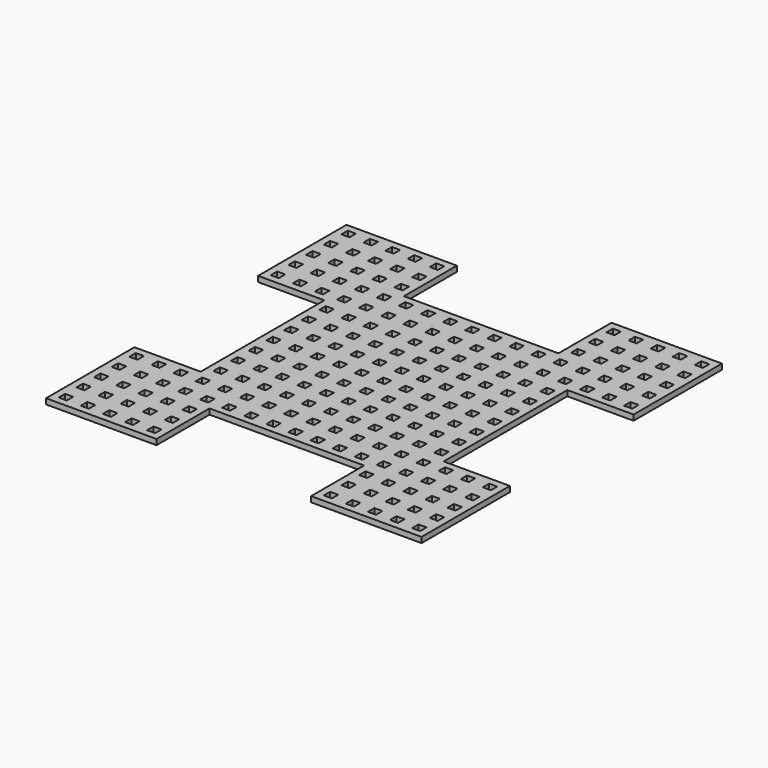
from build123d import *

# Parameters (mm, degrees)
F0_W     = 4.6228
F0_H     = 4.6228
F1_DEPTH = 3.175


# Not quite as in the source:
# - a length typed as a fraction of an inch, garbled in the dataset ("3 / 203.2 mm" for 3/8 in), is restored


with BuildPart() as f1:
    # F0 (on Top) → F1 (new body)
    with BuildSketch(Plane.XY):
        Polygon((114.3, 101.6), (101.6, 101.6), (50.8, 101.6), (50.8, 63.5), (-38.1, 63.5), (-38.1, 101.6), (-95.25, 101.6), (-101.6, 101.6), (-101.6, 95.25), (-101.6, 38.1), (-63.5, 38.1), (-63.5, -50.8), (-101.6, -50.8), (-101.6, -114.3), (-38.1, -114.3), (-38.1, -76.2), (50.8, -76.2), (50.8, -114.3), (114.3, -114.3), (114.3, -50.8), (76.2, -50.8), (76.2, 38.1), (114.3, 38.1), align=None)
        with Locations((-95.25, -107.95)):
            Rectangle(F0_W, F0_H, mode=Mode.SUBTRACT)
        with Locations((-82.55, -107.95)):
            Rectangle(F0_W, F0_H, mode=Mode.SUBTRACT)
        with Locations((-95.25, -95.25)):
            Rectangle(F0_W, F0_H, mode=Mode.SUBTRACT)
        with Locations((-82.55, -95.25)):
            Rectangle(F0_W, F0_H, mode=Mode.SUBTRACT)
        with Locations((-69.85, -107.95)):
            Rectangle(F0_W, F0_H, mode=Mode.SUBTRACT)
        with Locations((-57.15, -107.95)):
            Rectangle(F0_W, F0_H, mode=Mode.SUBTRACT)
        with Locations((-69.85, -95.25)):
            Rectangle(F0_W, F0_H, mode=Mode.SUBTRACT)
        with Locations((-57.15, -95.25)):
            Rectangle(F0_W, F0_H, mode=Mode.SUBTRACT)
        with Locations((-95.25, -82.55)):
            Rectangle(F0_W, F0_H, mode=Mode.SUBTRACT)
        with Locations((-82.55, -82.55)):
            Rectangle(F0_W, F0_H, mode=Mode.SUBTRACT)
        with Locations((-95.25, -69.85)):
            Rectangle(F0_W, F0_H, mode=Mode.SUBTRACT)
        with Locations((-82.55, -69.85)):
            Rectangle(F0_W, F0_H, mode=Mode.SUBTRACT)
        with Locations((-69.85, -82.55)):
            Rectangle(F0_W, F0_H, mode=Mode.SUBTRACT)
        with Locations((-57.15, -82.55)):
            Rectangle(F0_W, F0_H, mode=Mode.SUBTRACT)
        with Locations((-69.85, -69.85)):
            Rectangle(F0_W, F0_H, mode=Mode.SUBTRACT)
        with Locations((-57.15, -69.85)):
            Rectangle(F0_W, F0_H, mode=Mode.SUBTRACT)
        with Locations((-44.45, -107.95)):
            Rectangle(F0_W, F0_H, mode=Mode.SUBTRACT)
        with Locations((-44.45, -95.25)):
            Rectangle(F0_W, F0_H, mode=Mode.SUBTRACT)
        with Locations((-44.45, -82.55)):
            Rectangle(F0_W, F0_H, mode=Mode.SUBTRACT)
        with Locations((-44.45, -69.85)):
            Rectangle(F0_W, F0_H, mode=Mode.SUBTRACT)
        with Locations((-31.75, -69.85)):
            Rectangle(F0_W, F0_H, mode=Mode.SUBTRACT)
        with Locations((-19.05, -69.85)):
            Rectangle(F0_W, F0_H, mode=Mode.SUBTRACT)
        with Locations((-6.35, -69.85)):
            Rectangle(F0_W, F0_H, mode=Mode.SUBTRACT)
        with Locations((-95.25, -57.15)):
            Rectangle(F0_W, F0_H, mode=Mode.SUBTRACT)
        with Locations((-82.55, -57.15)):
            Rectangle(F0_W, F0_H, mode=Mode.SUBTRACT)
        with Locations((-69.85, -57.15)):
            Rectangle(F0_W, F0_H, mode=Mode.SUBTRACT)
        with Locations((-57.15, -57.15)):
            Rectangle(F0_W, F0_H, mode=Mode.SUBTRACT)
        with Locations((-57.15, -44.45)):
            Rectangle(F0_W, F0_H, mode=Mode.SUBTRACT)
        with Locations((-57.15, -31.75)):
            Rectangle(F0_W, F0_H, mode=Mode.SUBTRACT)
        with Locations((-57.15, -19.05)):
            Rectangle(F0_W, F0_H, mode=Mode.SUBTRACT)
        with Locations((-44.45, -57.15)):
            Rectangle(F0_W, F0_H, mode=Mode.SUBTRACT)
        with Locations((-31.75, -57.15)):
            Rectangle(F0_W, F0_H, mode=Mode.SUBTRACT)
        with Locations((-44.45, -44.45)):
            Rectangle(F0_W, F0_H, mode=Mode.SUBTRACT)
        with Locations((-31.75, -44.45)):
            Rectangle(F0_W, F0_H, mode=Mode.SUBTRACT)
        with Locations((-19.05, -57.15)):
            Rectangle(F0_W, F0_H, mode=Mode.SUBTRACT)
        with Locations((-6.35, -57.15)):
            Rectangle(F0_W, F0_H, mode=Mode.SUBTRACT)
        with Locations((-19.05, -44.45)):
            Rectangle(F0_W, F0_H, mode=Mode.SUBTRACT)
        with Locations((-6.35, -44.45)):
            Rectangle(F0_W, F0_H, mode=Mode.SUBTRACT)
        with Locations((-44.45, -31.75)):
            Rectangle(F0_W, F0_H, mode=Mode.SUBTRACT)
        with Locations((-31.75, -31.75)):
            Rectangle(F0_W, F0_H, mode=Mode.SUBTRACT)
        with Locations((-44.45, -19.05)):
            Rectangle(F0_W, F0_H, mode=Mode.SUBTRACT)
        with Locations((-31.75, -19.05)):
            Rectangle(F0_W, F0_H, mode=Mode.SUBTRACT)
        with Locations((-19.05, -31.75)):
            Rectangle(F0_W, F0_H, mode=Mode.SUBTRACT)
        with Locations((-6.35, -31.75)):
            Rectangle(F0_W, F0_H, mode=Mode.SUBTRACT)
        with Locations((-19.05, -19.05)):
            Rectangle(F0_W, F0_H, mode=Mode.SUBTRACT)
        with Locations((-6.35, -19.05)):
            Rectangle(F0_W, F0_H, mode=Mode.SUBTRACT)
        with Locations((57.15, -107.95)):
            Rectangle(F0_W, F0_H, mode=Mode.SUBTRACT)
        with Locations((57.15, -95.25)):
            Rectangle(F0_W, F0_H, mode=Mode.SUBTRACT)
        with Locations((6.35, -69.85)):
            Rectangle(F0_W, F0_H, mode=Mode.SUBTRACT)
        with Locations((19.05, -69.85)):
            Rectangle(F0_W, F0_H, mode=Mode.SUBTRACT)
        with Locations((31.75, -69.85)):
            Rectangle(F0_W, F0_H, mode=Mode.SUBTRACT)
        with Locations((57.15, -82.55)):
            Rectangle(F0_W, F0_H, mode=Mode.SUBTRACT)
        with Locations((44.45, -69.85)):
            Rectangle(F0_W, F0_H, mode=Mode.SUBTRACT)
        with Locations((57.15, -69.85)):
            Rectangle(F0_W, F0_H, mode=Mode.SUBTRACT)
        with Locations((69.85, -107.95)):
            Rectangle(F0_W, F0_H, mode=Mode.SUBTRACT)
        with Locations((82.55, -107.95)):
            Rectangle(F0_W, F0_H, mode=Mode.SUBTRACT)
        with Locations((69.85, -95.25)):
            Rectangle(F0_W, F0_H, mode=Mode.SUBTRACT)
        with Locations((82.55, -95.25)):
            Rectangle(F0_W, F0_H, mode=Mode.SUBTRACT)
        with Locations((95.25, -107.95)):
            Rectangle(F0_W, F0_H, mode=Mode.SUBTRACT)
        with Locations((107.95, -107.95)):
            Rectangle(F0_W, F0_H, mode=Mode.SUBTRACT)
        with Locations((95.25, -95.25)):
            Rectangle(F0_W, F0_H, mode=Mode.SUBTRACT)
        with Locations((107.95, -95.25)):
            Rectangle(F0_W, F0_H, mode=Mode.SUBTRACT)
        with Locations((69.85, -82.55)):
            Rectangle(F0_W, F0_H, mode=Mode.SUBTRACT)
        with Locations((82.55, -82.55)):
            Rectangle(F0_W, F0_H, mode=Mode.SUBTRACT)
        with Locations((69.85, -69.85)):
            Rectangle(F0_W, F0_H, mode=Mode.SUBTRACT)
        with Locations((82.55, -69.85)):
            Rectangle(F0_W, F0_H, mode=Mode.SUBTRACT)
        with Locations((95.25, -82.55)):
            Rectangle(F0_W, F0_H, mode=Mode.SUBTRACT)
        with Locations((107.95, -82.55)):
            Rectangle(F0_W, F0_H, mode=Mode.SUBTRACT)
        with Locations((95.25, -69.85)):
            Rectangle(F0_W, F0_H, mode=Mode.SUBTRACT)
        with Locations((107.95, -69.85)):
            Rectangle(F0_W, F0_H, mode=Mode.SUBTRACT)
        with Locations((6.35, -57.15)):
            Rectangle(F0_W, F0_H, mode=Mode.SUBTRACT)
        with Locations((19.05, -57.15)):
            Rectangle(F0_W, F0_H, mode=Mode.SUBTRACT)
        with Locations((31.75, -57.15)):
            Rectangle(F0_W, F0_H, mode=Mode.SUBTRACT)
        with Locations((6.35, -44.45)):
            Rectangle(F0_W, F0_H, mode=Mode.SUBTRACT)
        with Locations((19.05, -44.45)):
            Rectangle(F0_W, F0_H, mode=Mode.SUBTRACT)
        with Locations((31.75, -44.45)):
            Rectangle(F0_W, F0_H, mode=Mode.SUBTRACT)
        with Locations((44.45, -57.15)):
            Rectangle(F0_W, F0_H, mode=Mode.SUBTRACT)
        with Locations((57.15, -57.15)):
            Rectangle(F0_W, F0_H, mode=Mode.SUBTRACT)
        with Locations((44.45, -44.45)):
            Rectangle(F0_W, F0_H, mode=Mode.SUBTRACT)
        with Locations((57.15, -44.45)):
            Rectangle(F0_W, F0_H, mode=Mode.SUBTRACT)
        with Locations((6.35, -31.75)):
            Rectangle(F0_W, F0_H, mode=Mode.SUBTRACT)
        with Locations((19.05, -31.75)):
            Rectangle(F0_W, F0_H, mode=Mode.SUBTRACT)
        with Locations((31.75, -31.75)):
            Rectangle(F0_W, F0_H, mode=Mode.SUBTRACT)
        with Locations((6.35, -19.05)):
            Rectangle(F0_W, F0_H, mode=Mode.SUBTRACT)
        with Locations((19.05, -19.05)):
            Rectangle(F0_W, F0_H, mode=Mode.SUBTRACT)
        with Locations((31.75, -19.05)):
            Rectangle(F0_W, F0_H, mode=Mode.SUBTRACT)
        with Locations((44.45, -31.75)):
            Rectangle(F0_W, F0_H, mode=Mode.SUBTRACT)
        with Locations((57.15, -31.75)):
            Rectangle(F0_W, F0_H, mode=Mode.SUBTRACT)
        with Locations((44.45, -19.05)):
            Rectangle(F0_W, F0_H, mode=Mode.SUBTRACT)
        with Locations((57.15, -19.05)):
            Rectangle(F0_W, F0_H, mode=Mode.SUBTRACT)
        with Locations((69.85, -57.15)):
            Rectangle(F0_W, F0_H, mode=Mode.SUBTRACT)
        with Locations((82.55, -57.15)):
            Rectangle(F0_W, F0_H, mode=Mode.SUBTRACT)
        with Locations((69.85, -44.45)):
            Rectangle(F0_W, F0_H, mode=Mode.SUBTRACT)
        with Locations((95.25, -57.15)):
            Rectangle(F0_W, F0_H, mode=Mode.SUBTRACT)
        with Locations((107.95, -57.15)):
            Rectangle(F0_W, F0_H, mode=Mode.SUBTRACT)
        with Locations((69.85, -31.75)):
            Rectangle(F0_W, F0_H, mode=Mode.SUBTRACT)
        with Locations((69.85, -19.05)):
            Rectangle(F0_W, F0_H, mode=Mode.SUBTRACT)
        with Locations((-57.15, -6.35)):
            Rectangle(F0_W, F0_H, mode=Mode.SUBTRACT)
        with Locations((-57.15, 6.35)):
            Rectangle(F0_W, F0_H, mode=Mode.SUBTRACT)
        with Locations((-57.15, 19.05)):
            Rectangle(F0_W, F0_H, mode=Mode.SUBTRACT)
        with Locations((-95.25, 44.45)):
            Rectangle(F0_W, F0_H, mode=Mode.SUBTRACT)
        with Locations((-82.55, 44.45)):
            Rectangle(F0_W, F0_H, mode=Mode.SUBTRACT)
        with Locations((-57.15, 31.75)):
            Rectangle(F0_W, F0_H, mode=Mode.SUBTRACT)
        with Locations((-69.85, 44.45)):
            Rectangle(F0_W, F0_H, mode=Mode.SUBTRACT)
        with Locations((-57.15, 44.45)):
            Rectangle(F0_W, F0_H, mode=Mode.SUBTRACT)
        with Locations((-44.45, -6.35)):
            Rectangle(F0_W, F0_H, mode=Mode.SUBTRACT)
        with Locations((-44.45, 6.35)):
            Rectangle(F0_W, F0_H, mode=Mode.SUBTRACT)
        with Locations((-31.75, -6.35)):
            Rectangle(F0_W, F0_H, mode=Mode.SUBTRACT)
        with Locations((-31.75, 6.35)):
            Rectangle(F0_W, F0_H, mode=Mode.SUBTRACT)
        with Locations((-44.45, 19.05)):
            Rectangle(F0_W, F0_H, mode=Mode.SUBTRACT)
        with Locations((-31.75, 19.05)):
            Rectangle(F0_W, F0_H, mode=Mode.SUBTRACT)
        with Locations((-19.05, -6.35)):
            Rectangle(F0_W, F0_H, mode=Mode.SUBTRACT)
        with Locations((-19.05, 6.35)):
            Rectangle(F0_W, F0_H, mode=Mode.SUBTRACT)
        with Locations((-6.35, -6.35)):
            Rectangle(F0_W, F0_H, mode=Mode.SUBTRACT)
        with Locations((-6.35, 6.35)):
            Rectangle(F0_W, F0_H, mode=Mode.SUBTRACT)
        with Locations((-19.05, 19.05)):
            Rectangle(F0_W, F0_H, mode=Mode.SUBTRACT)
        with Locations((-6.35, 19.05)):
            Rectangle(F0_W, F0_H, mode=Mode.SUBTRACT)
        with Locations((-44.45, 31.75)):
            Rectangle(F0_W, F0_H, mode=Mode.SUBTRACT)
        with Locations((-31.75, 31.75)):
            Rectangle(F0_W, F0_H, mode=Mode.SUBTRACT)
        with Locations((-44.45, 44.45)):
            Rectangle(F0_W, F0_H, mode=Mode.SUBTRACT)
        with Locations((-31.75, 44.45)):
            Rectangle(F0_W, F0_H, mode=Mode.SUBTRACT)
        with Locations((-19.05, 31.75)):
            Rectangle(F0_W, F0_H, mode=Mode.SUBTRACT)
        with Locations((-6.35, 31.75)):
            Rectangle(F0_W, F0_H, mode=Mode.SUBTRACT)
        with Locations((-19.05, 44.45)):
            Rectangle(F0_W, F0_H, mode=Mode.SUBTRACT)
        with Locations((-6.35, 44.45)):
            Rectangle(F0_W, F0_H, mode=Mode.SUBTRACT)
        with Locations((-95.25, 57.15)):
            Rectangle(F0_W, F0_H, mode=Mode.SUBTRACT)
        with Locations((-82.55, 57.15)):
            Rectangle(F0_W, F0_H, mode=Mode.SUBTRACT)
        with Locations((-95.25, 69.85)):
            Rectangle(F0_W, F0_H, mode=Mode.SUBTRACT)
        with Locations((-82.55, 69.85)):
            Rectangle(F0_W, F0_H, mode=Mode.SUBTRACT)
        with Locations((-69.85, 57.15)):
            Rectangle(F0_W, F0_H, mode=Mode.SUBTRACT)
        with Locations((-57.15, 57.15)):
            Rectangle(F0_W, F0_H, mode=Mode.SUBTRACT)
        with Locations((-69.85, 69.85)):
            Rectangle(F0_W, F0_H, mode=Mode.SUBTRACT)
        with Locations((-57.15, 69.85)):
            Rectangle(F0_W, F0_H, mode=Mode.SUBTRACT)
        with Locations((-95.25, 82.55)):
            Rectangle(F0_W, F0_H, mode=Mode.SUBTRACT)
        with Locations((-82.55, 82.55)):
            Rectangle(F0_W, F0_H, mode=Mode.SUBTRACT)
        with Locations((-95.25, 95.25)):
            Rectangle(F0_W, F0_H, mode=Mode.SUBTRACT)
        with Locations((-82.55, 95.25)):
            Rectangle(F0_W, F0_H, mode=Mode.SUBTRACT)
        with Locations((-69.85, 82.55)):
            Rectangle(F0_W, F0_H, mode=Mode.SUBTRACT)
        with Locations((-57.15, 82.55)):
            Rectangle(F0_W, F0_H, mode=Mode.SUBTRACT)
        with Locations((-69.85, 95.25)):
            Rectangle(F0_W, F0_H, mode=Mode.SUBTRACT)
        with Locations((-57.15, 95.25)):
            Rectangle(F0_W, F0_H, mode=Mode.SUBTRACT)
        with Locations((-44.45, 57.15)):
            Rectangle(F0_W, F0_H, mode=Mode.SUBTRACT)
        with Locations((-31.75, 57.15)):
            Rectangle(F0_W, F0_H, mode=Mode.SUBTRACT)
        with Locations((-44.45, 69.85)):
            Rectangle(F0_W, F0_H, mode=Mode.SUBTRACT)
        with Locations((-19.05, 57.15)):
            Rectangle(F0_W, F0_H, mode=Mode.SUBTRACT)
        with Locations((-6.35, 57.15)):
            Rectangle(F0_W, F0_H, mode=Mode.SUBTRACT)
        with Locations((-44.45, 82.55)):
            Rectangle(F0_W, F0_H, mode=Mode.SUBTRACT)
        with Locations((-44.45, 95.25)):
            Rectangle(F0_W, F0_H, mode=Mode.SUBTRACT)
        with Locations((6.35, -6.35)):
            Rectangle(F0_W, F0_H, mode=Mode.SUBTRACT)
        with Locations((19.05, -6.35)):
            Rectangle(F0_W, F0_H, mode=Mode.SUBTRACT)
        with Locations((6.35, 6.35)):
            Rectangle(F0_W, F0_H, mode=Mode.SUBTRACT)
        with Locations((19.05, 6.35)):
            Rectangle(F0_W, F0_H, mode=Mode.SUBTRACT)
        with Locations((31.75, -6.35)):
            Rectangle(F0_W, F0_H, mode=Mode.SUBTRACT)
        with Locations((31.75, 6.35)):
            Rectangle(F0_W, F0_H, mode=Mode.SUBTRACT)
        with Locations((6.35, 19.05)):
            Rectangle(F0_W, F0_H, mode=Mode.SUBTRACT)
        with Locations((19.05, 19.05)):
            Rectangle(F0_W, F0_H, mode=Mode.SUBTRACT)
        with Locations((31.75, 19.05)):
            Rectangle(F0_W, F0_H, mode=Mode.SUBTRACT)
        with Locations((44.45, -6.35)):
            Rectangle(F0_W, F0_H, mode=Mode.SUBTRACT)
        with Locations((44.45, 6.35)):
            Rectangle(F0_W, F0_H, mode=Mode.SUBTRACT)
        with Locations((57.15, -6.35)):
            Rectangle(F0_W, F0_H, mode=Mode.SUBTRACT)
        with Locations((57.15, 6.35)):
            Rectangle(F0_W, F0_H, mode=Mode.SUBTRACT)
        with Locations((44.45, 19.05)):
            Rectangle(F0_W, F0_H, mode=Mode.SUBTRACT)
        with Locations((57.15, 19.05)):
            Rectangle(F0_W, F0_H, mode=Mode.SUBTRACT)
        with Locations((6.35, 31.75)):
            Rectangle(F0_W, F0_H, mode=Mode.SUBTRACT)
        with Locations((19.05, 31.75)):
            Rectangle(F0_W, F0_H, mode=Mode.SUBTRACT)
        with Locations((31.75, 31.75)):
            Rectangle(F0_W, F0_H, mode=Mode.SUBTRACT)
        with Locations((6.35, 44.45)):
            Rectangle(F0_W, F0_H, mode=Mode.SUBTRACT)
        with Locations((19.05, 44.45)):
            Rectangle(F0_W, F0_H, mode=Mode.SUBTRACT)
        with Locations((31.75, 44.45)):
            Rectangle(F0_W, F0_H, mode=Mode.SUBTRACT)
        with Locations((44.45, 31.75)):
            Rectangle(F0_W, F0_H, mode=Mode.SUBTRACT)
        with Locations((57.15, 31.75)):
            Rectangle(F0_W, F0_H, mode=Mode.SUBTRACT)
        with Locations((44.45, 44.45)):
            Rectangle(F0_W, F0_H, mode=Mode.SUBTRACT)
        with Locations((57.15, 44.45)):
            Rectangle(F0_W, F0_H, mode=Mode.SUBTRACT)
        with Locations((69.85, -6.35)):
            Rectangle(F0_W, F0_H, mode=Mode.SUBTRACT)
        with Locations((69.85, 6.35)):
            Rectangle(F0_W, F0_H, mode=Mode.SUBTRACT)
        with Locations((69.85, 19.05)):
            Rectangle(F0_W, F0_H, mode=Mode.SUBTRACT)
        with Locations((69.85, 31.75)):
            Rectangle(F0_W, F0_H, mode=Mode.SUBTRACT)
        with Locations((69.85, 44.45)):
            Rectangle(F0_W, F0_H, mode=Mode.SUBTRACT)
        with Locations((82.55, 44.45)):
            Rectangle(F0_W, F0_H, mode=Mode.SUBTRACT)
        with Locations((95.25, 44.45)):
            Rectangle(F0_W, F0_H, mode=Mode.SUBTRACT)
        with Locations((107.95, 44.45)):
            Rectangle(F0_W, F0_H, mode=Mode.SUBTRACT)
        with Locations((6.35, 57.15)):
            Rectangle(F0_W, F0_H, mode=Mode.SUBTRACT)
        with Locations((19.05, 57.15)):
            Rectangle(F0_W, F0_H, mode=Mode.SUBTRACT)
        with Locations((31.75, 57.15)):
            Rectangle(F0_W, F0_H, mode=Mode.SUBTRACT)
        with Locations((44.45, 57.15)):
            Rectangle(F0_W, F0_H, mode=Mode.SUBTRACT)
        with Locations((57.15, 57.15)):
            Rectangle(F0_W, F0_H, mode=Mode.SUBTRACT)
        with Locations((57.15, 69.85)):
            Rectangle(F0_W, F0_H, mode=Mode.SUBTRACT)
        with Locations((57.15, 82.55)):
            Rectangle(F0_W, F0_H, mode=Mode.SUBTRACT)
        with Locations((57.15, 95.25)):
            Rectangle(F0_W, F0_H, mode=Mode.SUBTRACT)
        with Locations((69.85, 57.15)):
            Rectangle(F0_W, F0_H, mode=Mode.SUBTRACT)
        with Locations((82.55, 57.15)):
            Rectangle(F0_W, F0_H, mode=Mode.SUBTRACT)
        with Locations((69.85, 69.85)):
            Rectangle(F0_W, F0_H, mode=Mode.SUBTRACT)
        with Locations((82.55, 69.85)):
            Rectangle(F0_W, F0_H, mode=Mode.SUBTRACT)
        with Locations((95.25, 57.15)):
            Rectangle(F0_W, F0_H, mode=Mode.SUBTRACT)
        with Locations((107.95, 57.15)):
            Rectangle(F0_W, F0_H, mode=Mode.SUBTRACT)
        with Locations((95.25, 69.85)):
            Rectangle(F0_W, F0_H, mode=Mode.SUBTRACT)
        with Locations((107.95, 69.85)):
            Rectangle(F0_W, F0_H, mode=Mode.SUBTRACT)
        with Locations((69.85, 82.55)):
            Rectangle(F0_W, F0_H, mode=Mode.SUBTRACT)
        with Locations((82.55, 82.55)):
            Rectangle(F0_W, F0_H, mode=Mode.SUBTRACT)
        with Locations((69.85, 95.25)):
            Rectangle(F0_W, F0_H, mode=Mode.SUBTRACT)
        with Locations((82.55, 95.25)):
            Rectangle(F0_W, F0_H, mode=Mode.SUBTRACT)
        with Locations((95.25, 82.55)):
            Rectangle(F0_W, F0_H, mode=Mode.SUBTRACT)
        with Locations((107.95, 82.55)):
            Rectangle(F0_W, F0_H, mode=Mode.SUBTRACT)
        with Locations((95.25, 95.25)):
            Rectangle(F0_W, F0_H, mode=Mode.SUBTRACT)
        with Locations((107.95, 95.25)):
            Rectangle(F0_W, F0_H, mode=Mode.SUBTRACT)
    extrude(amount=F1_DEPTH)


solid = f1.part
